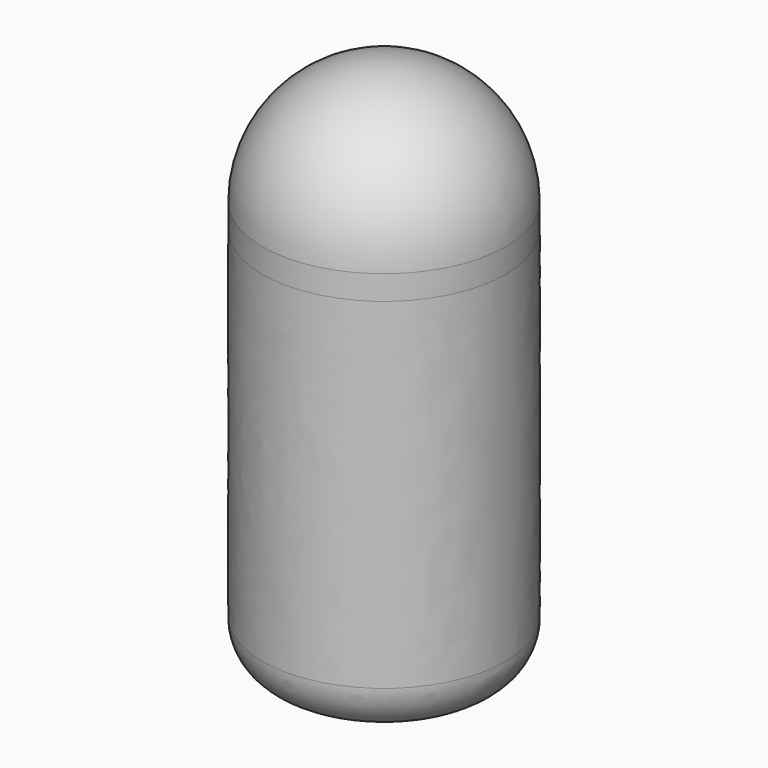
from build123d import *

# Parameters (mm, degrees)
F4_R  = 63.5
F2_R  = 63.5
F0_R  = 63.5
F6_R  = 25.4
F8_R  = 63.5
F10_R = 63.5


with BuildPart() as f5:
    # F4 (on offset) → F5 section 0
    with BuildSketch(Plane.XY.offset(203.2)):
        Circle(F4_R)
    # F2 (on offset) → F5 section 1
    with BuildSketch(Plane.XY.offset(101.6)):
        Circle(F2_R)
    # F0 (on Top) → F5 section 2
    with BuildSketch(Plane.XY):
        Circle(F0_R)
    loft()

    # F6
    f6_edges = [f5.edges().sort_by_distance(p)[0] for p in [
        (-63.5, 0, 0),
    ]]
    fillet(f6_edges, radius=F6_R)

    # F4 (on offset) → F9 section 0
    with BuildSketch(Plane.XY.offset(203.2)):
        Circle(F4_R)
    # F8 (on offset) → F9 section 1
    with BuildSketch(Plane.XY.offset(279.4)):
        Circle(F8_R)
    loft()

    # F10
    f10_edges = [f5.edges().sort_by_distance(p)[0] for p in [
        (-63.5, 0, 279.4),
    ]]
    fillet(f10_edges, radius=F10_R)


solid = f5.part
